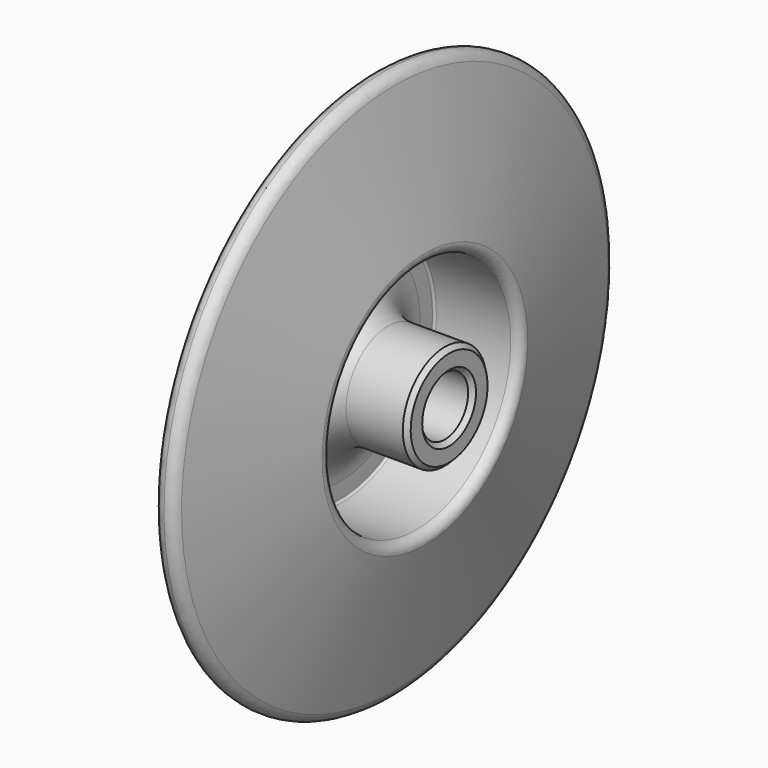
from build123d import *

# Parameters (mm, degrees)
F2_R    = 0.5
F3_R    = 2
F4_SIZE = 1
F5_R    = 11
F6_R    = 1.99999
F7_SIZE = 1
F8_R    = 2.49999
F9_R    = 5


# Not quite as in the source:
# - a fillet or chamfer is up to 0.001 mm smaller than in the source, because OpenCascade refuses the exact size


with BuildPart() as f1:
    # F0 (on Front) → F1 (revolve)
    with BuildSketch(Plane.XZ):
        with BuildLine():
            Line((0, 31), (0, 4.7))
            Line((0, 4.7), (8, 4.7))
            Line((8, 4.7), (8, 6.7))
            Line((8, 6.7), (33, 6.7))
            Line((33, 6.7), (33, 12))
            Line((33, 12), (8, 12))
            Line((8, 12), (8, 27))
            Line((8, 27), (28, 27))
            Line((28, 27), (20.118426236, 63))
            Line((20.118426236, 63), (15, 63))
            Line((15, 63), (22.0058433458, 31))
            Line((22.0058433458, 31), (6, 31))
            ThreePointArc((6, 31), (3, 34), (0, 31))
        make_face()
    revolve(axis=Axis((1.1409256999, 0, 0), (1, 0, 0)))

    # F2
    f2_edges = [f1.edges().sort_by_distance(p)[0] for p in [
        (8, 0, -27),
    ]]
    fillet(f2_edges, radius=F2_R)

    # F3
    f3_edges = [f1.edges().sort_by_distance(p)[0] for p in [
        (28, 0, -27),
    ]]
    fillet(f3_edges, radius=F3_R)

    # F4
    f4_edges = [f1.edges().sort_by_distance(p)[0] for p in [
        (33, 0, -6.7),
        (33, 0, -12),
    ]]
    chamfer(f4_edges, length=F4_SIZE)

    # F5
    f5_edges = [f1.edges().sort_by_distance(p)[0] for p in [
        (8, 0, -12),
    ]]
    fillet(f5_edges, radius=F5_R)

    # F6 (radius 2 in the source; OpenCascade refuses exactly that, so slightly less here)
    f6_edges = [f1.edges().sort_by_distance(p)[0] for p in [
        (8, 0, -6.7),
    ]]
    fillet(f6_edges, radius=F6_R)

    # F7
    f7_edges = [f1.edges().sort_by_distance(p)[0] for p in [
        (0, 0, -4.7),
    ]]
    chamfer(f7_edges, length=F7_SIZE)

    # F8 (radius 2.5 in the source; OpenCascade refuses exactly that, so slightly less here)
    f8_edges = [f1.edges().sort_by_distance(p)[0] for p in [
        (15, 0, -63),
        (20.118426, 0, -63),
    ]]
    fillet(f8_edges, radius=F8_R)

    # F9
    f9_edges = [f1.edges().sort_by_distance(p)[0] for p in [
        (22.005843, 0, -31),
    ]]
    fillet(f9_edges, radius=F9_R)


solid = f1.part
